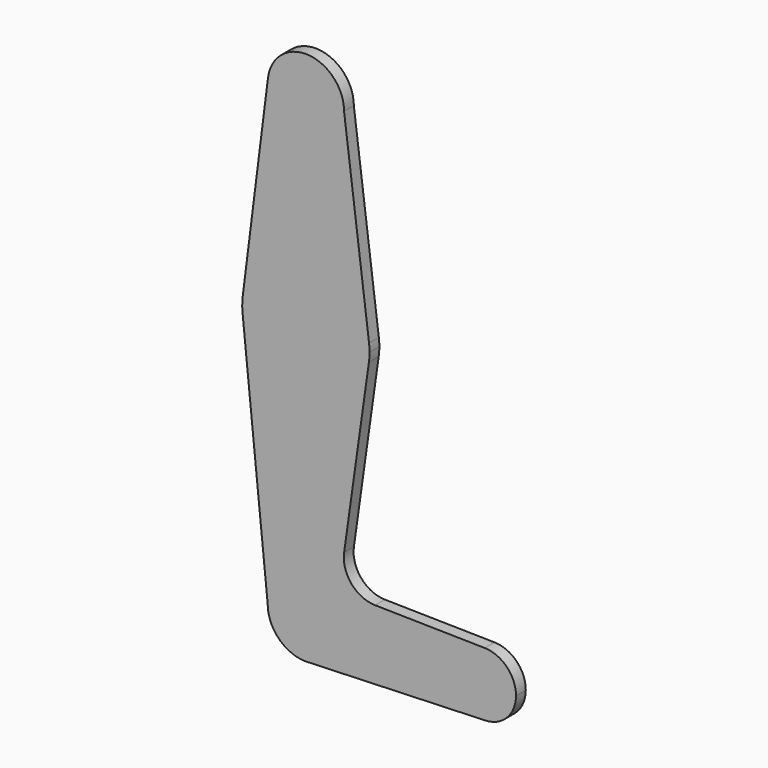
from build123d import *

# Parameters (mm, degrees)
F0_R     = 3.175
F1_DEPTH = 3.048


with BuildPart() as f1:
    # F0 (on Front) → F1 (new body)
    with BuildSketch(Plane.XZ):
        with BuildLine():
            ThreePointArc((9.525, 114.3), (0.596483242, 123.8063048942), (-9.4502929642, 115.490625))
            ThreePointArc((-9.4502929642, 115.490625), (-7.14375, 107.9998046905), (0, 104.775))
            ThreePointArc((0, 104.775), (6.7351920908, 107.5648079092), (9.525, 114.3))
        make_face()
        with BuildLine():
            ThreePointArc((3.175, 114.3), (2.2450640303, 112.0549359697), (0, 111.125))
            ThreePointArc((0, 111.125), (-2.2450640303, 116.5450640303), (3.175, 114.3))
        make_face(mode=Mode.SUBTRACT)
        with BuildLine():
            Line((0, 47.625), (0, 9.525))
            ThreePointArc((0, 9.525), (6.7351920908, 6.7351920908), (9.525, 0))
            Line((9.525, 0), (36.5125, 0))
            ThreePointArc((36.5125, 0), (38.8886909991, 5.663545572), (44.5945783487, 7.9361831727))
            Line((44.5945783487, 7.9361831727), (17.2606145929, 8.4341428668))
            ThreePointArc((17.2606145929, 8.4341428668), (11.3562252192, 11.224257518), (9.5333913565, 17.4951290964))
            Line((9.5333913565, 17.4951290964), (15.7189155447, 61.2793426425))
            ThreePointArc((15.7189155447, 61.2793426425), (10.4106361345, 51.5152480094), (0, 47.625))
        make_face()
        with BuildLine():
            ThreePointArc((-15.7942028036, 61.9003804205), (-10.644756084, 51.722700101), (0, 47.625))
            Line((0, 47.625), (0, 60.325))
            ThreePointArc((0, 60.325), (-3.175, 63.5), (0, 66.675))
            Line((0, 66.675), (0, 79.375))
            ThreePointArc((0, 79.375), (-10.5003255158, 75.40625), (-15.7504882737, 65.484375))
            ThreePointArc((-15.7504882737, 65.484375), (-15.8738192656, 63.6936154008), (-15.7942028036, 61.9003804205))
        make_face()
        with BuildLine():
            Line((0, 100.0252), (0, 79.375))
            ThreePointArc((0, 79.375), (10.4912828548, 75.4142187767), (15.7474569047, 65.5082893304))
            Line((15.7474569047, 65.5082893304), (9.525, 114.3))
            ThreePointArc((9.525, 114.3), (6.7351920908, 107.5648079092), (0, 104.775))
            Line((0, 104.775), (0, 100.0252))
        make_face()
        with BuildLine():
            ThreePointArc((44.5945783487, 7.9361831727), (38.8886909991, 5.663545572), (36.5125, 0))
            ThreePointArc((36.5125, 0), (38.9380895153, -5.7116327839), (44.7324052746, -7.9324746146))
            ThreePointArc((44.7324052746, -7.9324746146), (50.1616327839, -5.5119104847), (52.3875, 0))
            ThreePointArc((52.3875, 0), (50.113545572, 5.5613090009), (44.5945783487, 7.9361831727))
        make_face()
        with BuildLine():
            ThreePointArc((47.625, 0), (44.45, -3.175), (41.275, 0))
            ThreePointArc((41.275, 0), (44.45, 3.175), (47.625, 0))
        make_face(mode=Mode.SUBTRACT)
        with BuildLine():
            Line((-9.4502929642, 115.490625), (-15.7504882737, 65.484375))
            ThreePointArc((-15.7504882737, 65.484375), (-10.5003255158, 75.40625), (0, 79.375))
            Line((0, 79.375), (0, 100.0252))
            Line((0, 100.0252), (0, 104.775))
            ThreePointArc((0, 104.775), (-7.14375, 107.9998046905), (-9.4502929642, 115.490625))
        make_face()
        with Locations((-3.175, 100.0252)):
            Circle(F0_R, mode=Mode.SUBTRACT)
        with BuildLine():
            Line((0, 60.325), (0, 47.625))
            ThreePointArc((0, 47.625), (10.4106361345, 51.5152480094), (15.7189155447, 61.2793426425))
            ThreePointArc((15.7189155447, 61.2793426425), (15.8359308105, 62.3869320038), (15.875, 63.5))
            ThreePointArc((15.875, 63.5), (15.8430821396, 64.5061676396), (15.7474569047, 65.5082893304))
            ThreePointArc((15.7474569047, 65.5082893304), (10.4912828548, 75.4142187767), (0, 79.375))
            Line((0, 79.375), (0, 66.675))
            ThreePointArc((0, 66.675), (2.2450640303, 65.7450640303), (3.175, 63.5))
            ThreePointArc((3.175, 63.5), (2.2450640303, 61.2549359697), (0, 60.325))
        make_face()
        with BuildLine():
            ThreePointArc((3.175, 0), (-2.2450640303, -2.2450640303), (0, 3.175))
            Line((0, 3.175), (0, 9.525))
            ThreePointArc((0, 9.525), (-6.7351920908, 6.7351920908), (-9.525, 0))
            ThreePointArc((-9.525, 0), (-6.7351920908, -6.7351920908), (0, -9.525))
            Line((0, -9.525), (0.6773435479, -9.500885786))
            ThreePointArc((0.6773435479, -9.500885786), (6.9705567315, -6.4912990883), (9.525, 0))
            Line((9.525, 0), (3.175, 0))
        make_face()
        with BuildLine():
            Line((36.5125, 0), (9.525, 0))
            ThreePointArc((9.525, 0), (6.9705567315, -6.4912990883), (0.6773435479, -9.500885786))
            Line((0.6773435479, -9.500885786), (44.7324052746, -7.9324746146))
            ThreePointArc((44.7324052746, -7.9324746146), (38.9380895153, -5.7116327839), (36.5125, 0))
        make_face()
        with BuildLine():
            ThreePointArc((-9.525, 0), (-6.7351920908, 6.7351920908), (0, 9.525))
            Line((0, 9.525), (0, 47.625))
            ThreePointArc((0, 47.625), (-10.644756084, 51.722700101), (-15.7942028036, 61.9003804205))
            Line((-15.7942028036, 61.9003804205), (-9.525, 0))
        make_face()
        with BuildLine():
            Line((0, 9.525), (0, 3.175))
            ThreePointArc((0, 3.175), (2.2450640303, 2.2450640303), (3.175, 0))
            Line((3.175, 0), (9.525, 0))
            ThreePointArc((9.525, 0), (6.7351920908, 6.7351920908), (0, 9.525))
        make_face()
        with BuildLine():
            ThreePointArc((0, -9.525), (0.3388863295, -9.5189695375), (0.6773435479, -9.500885786))
            Line((0.6773435479, -9.500885786), (0, -9.525))
        make_face()
        with BuildLine():
            ThreePointArc((3.175, 114.3), (-2.2450640303, 116.5450640303), (0, 111.125))
            ThreePointArc((0, 111.125), (2.2450640303, 112.0549359697), (3.175, 114.3))
        make_face()
        with BuildLine():
            ThreePointArc((47.625, 0), (44.45, 3.175), (41.275, 0))
            ThreePointArc((41.275, 0), (44.45, -3.175), (47.625, 0))
        make_face()
        with Locations((-3.175, 100.0252)):
            Circle(F0_R)
        with BuildLine():
            ThreePointArc((0, 66.675), (-3.175, 63.5), (0, 60.325))
            Line((0, 60.325), (0, 63.5))
            Line((0, 63.5), (0, 66.675))
        make_face()
        with BuildLine():
            Line((0, 63.5), (0, 60.325))
            ThreePointArc((0, 60.325), (2.2450640303, 61.2549359697), (3.175, 63.5))
            ThreePointArc((3.175, 63.5), (2.2450640303, 65.7450640303), (0, 66.675))
            Line((0, 66.675), (0, 63.5))
        make_face()
        with BuildLine():
            Line((0, 3.175), (0, 0))
            Line((0, 0), (3.175, 0))
            ThreePointArc((3.175, 0), (2.2450640303, 2.2450640303), (0, 3.175))
        make_face()
        with BuildLine():
            Line((3.175, 0), (0, 0))
            Line((0, 0), (0, 3.175))
            ThreePointArc((0, 3.175), (-2.2450640303, -2.2450640303), (3.175, 0))
        make_face()
    extrude(amount=F1_DEPTH)


solid = f1.part
